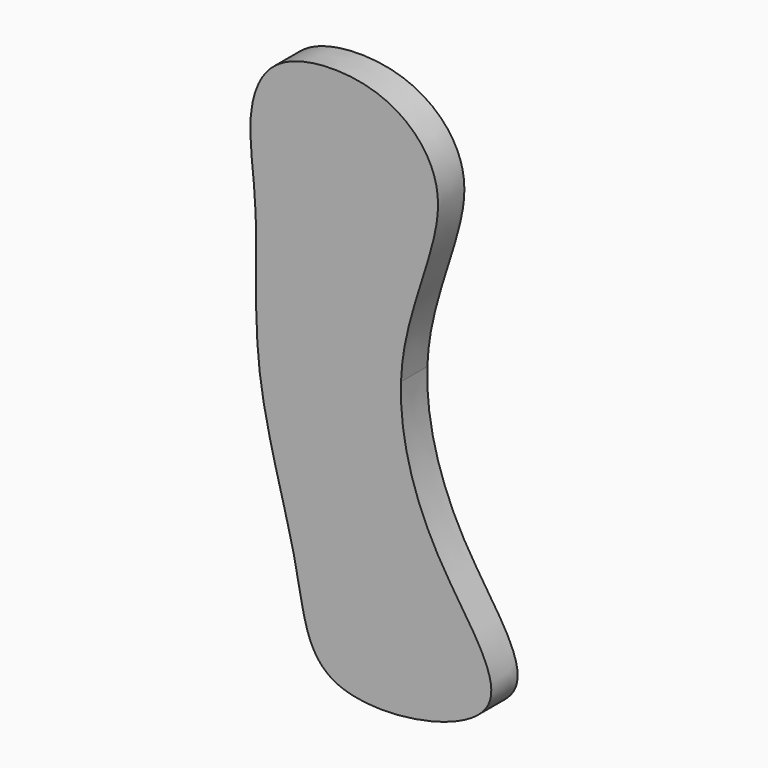
from build123d import *

# Parameters (mm, degrees)
F1_DEPTH = 8.382


with BuildPart() as f1:
    # F0 (on Front) → F1 (new body)
    with BuildSketch(Plane.XZ):
        with BuildLine():
            add(Edge.make_bspline(
                [(-29.6290591359, 52.0929135382), (-29.1721656164, 57.2353658162), (-25.3808979719, 67.8252387617), (-4.7281024672, 70.6918550098), (11.8342986189, 64.4966971157), (22.6536969715, 46.4422673983), (10.0123512504, 22.2982985007), (8.6612392429, 6.7797701254), (8.5913060935, 4.8405602013)],
                knots=[0, 0, 0, 0, 0.0605711944, 0.1290669119, 0.1946194996, 0.2603741999, 0.358065015, 0.3720069572, 0.3720069572, 0.3720069572, 0.3720069572], degree=3))
            add(Edge.make_bspline(
                [(8.5913060935, 4.8405602013), (8.1325491937, -7.8805304521), (15.5879350635, -32.9745869754), (45.4305166994, -65.3564264611), (-14.8203768574, -75.9854083707), (-16.7404311733, -43.9916462979), (-30.165620113, -6.1015732313), (-27.1133502841, 31.1983059283), (-30.1669803996, 46.0384734785), (-29.6290591359, 52.0929135382)],
                knots=[0.3720069572, 0.3720069572, 0.3720069572, 0.3720069572, 0.4634651891, 0.551761892, 0.650000246, 0.7292991273, 0.8318480954, 0.928686812, 1, 1, 1, 1], degree=3))
        make_face()
    extrude(amount=F1_DEPTH)


solid = f1.part
